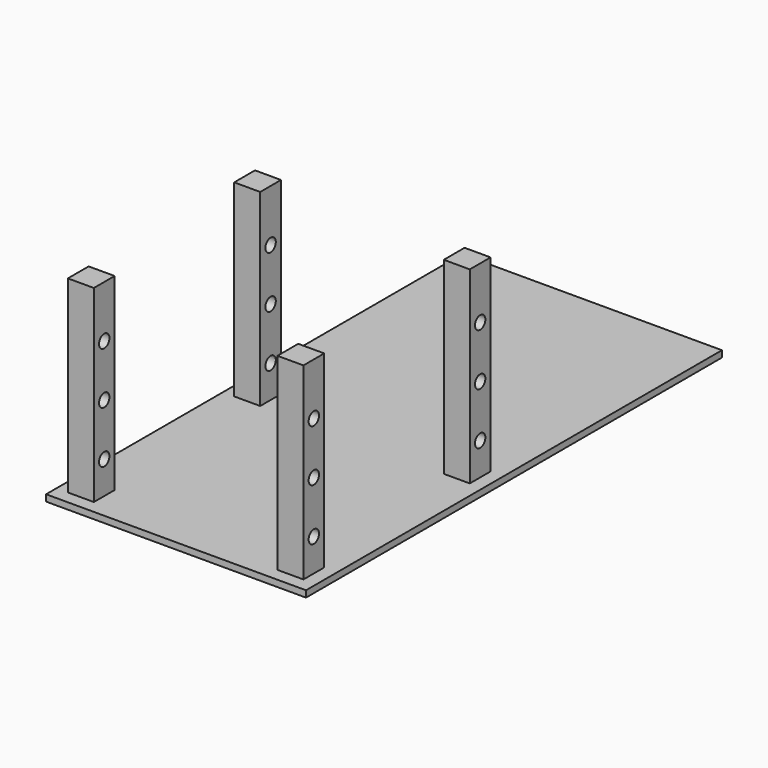
from build123d import *

# Parameters (mm, degrees)
F0_W     = 1000
F0_H     = 2000
F1_DEPTH = 25
F3_W     = 100
F3_H     = 725
F3_R     = 25
F4_DEPTH = 100


# Not quite as in the source:
# - a pattern or mirror of a feature is missing from the dataset's text; its kind, count and spacing are read off the source's solid


with BuildPart() as f1:
    # F0 (on Top) → F1 (new body)
    with BuildSketch(Plane.XY):
        with Locations((3.129221499, -3.3162072057)):
            Rectangle(F0_W, F0_H)
    extrude(amount=F1_DEPTH)

    # F3 (on offset) → F4 (join)
    with BuildSketch(Plane.YZ.offset(453.129221499)):
        with Locations((-903.3162072057, 387.5)):
            Rectangle(F3_W, F3_H)
        with Locations((-903.3162072057, 150)):
            Circle(F3_R, mode=Mode.SUBTRACT)
        with Locations((-903.3162072057, 350)):
            Circle(F3_R, mode=Mode.SUBTRACT)
        with Locations((-903.3162072057, 550)):
            Circle(F3_R, mode=Mode.SUBTRACT)
        with Locations((-103.3162072057, 387.5)):
            Rectangle(F3_W, F3_H)
        with Locations((-103.3162072057, 150)):
            Circle(F3_R, mode=Mode.SUBTRACT)
        with Locations((-103.3162072057, 350)):
            Circle(F3_R, mode=Mode.SUBTRACT)
        with Locations((-103.3162072057, 550)):
            Circle(F3_R, mode=Mode.SUBTRACT)
    f4 = extrude(amount=-F4_DEPTH)

    # F4_copies: F4 across plane
    add(f4.mirror(Plane(origin=(0, 0, 0), x_dir=(0, 0, -1), z_dir=(-1, 0, 0))))


solid = f1.part
